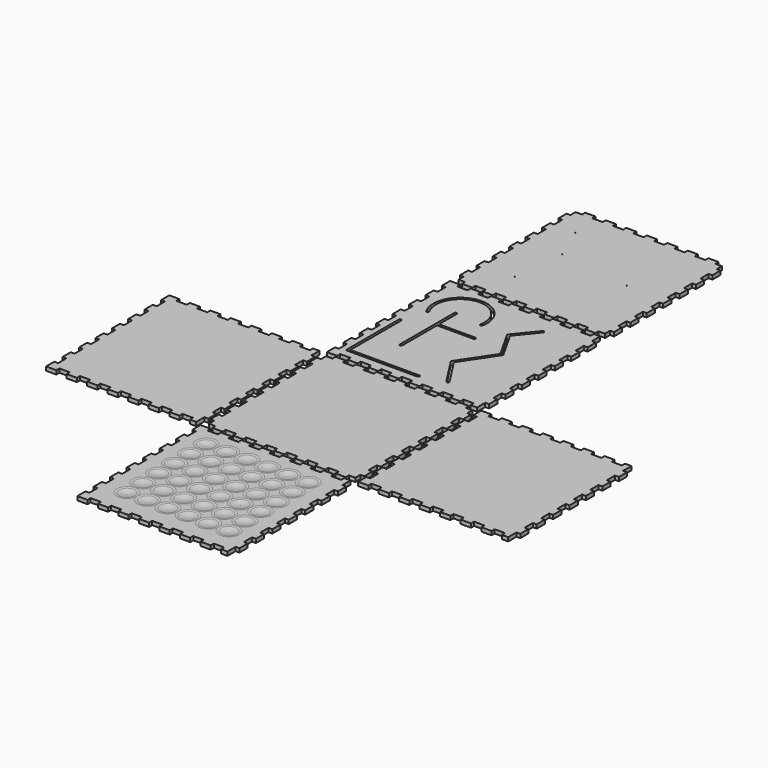
from build123d import *

# Parameters (mm, degrees)
F1_DEPTH = 19.05
F3_DEPTH = 19.051
F4_R     = 44.1721582368
F5_DEPTH = 6.35
F7_R     = 45.72
F8_R     = 1.27
F9_DEPTH = 19.051


# Not quite as in the source:
# - a fillet or chamfer that OpenCascade refuses, or shapes differently, is made with other operations: its cross-section is extruded or revolved along the edge and cut away or added
# - a feature names something its author has since deleted; it is built from what else it names


with BuildPart() as f1:
    # F0 (on Top) → F1 (new body)
    with BuildSketch(Plane.XY):
        Polygon((-361.9498222, 827.8001224), (-361.9498222, 796.0501224), (-330.1998222, 796.0501224), (-330.1998222, 777.0001224), (-279.3998222, 777.0001224), (-279.3998222, 796.0501224), (-228.5998222, 796.0501224), (-228.5998222, 777.0001224), (-177.7998222, 777.0001224), (-177.7998222, 796.0501224), (-126.9998222, 796.0501224), (-126.9998222, 777.0001224), (-76.1998222, 777.0001224), (-76.1998222, 796.0501224), (-25.3998222, 796.0501224), (-25.3998222, 777.0001224), (25.4001778, 777.0001224), (25.4001778, 796.0501224), (76.2001778, 796.0501224), (76.2001778, 777.0001224), (127.0001778, 777.0001224), (127.0001778, 796.0501224), (177.8001778, 796.0501224), (177.8001778, 777.0001224), (228.6001778, 777.0001224), (228.6001778, 796.0501224), (279.4001778, 796.0501224), (279.4001778, 777.0001224), (330.2001778, 777.0001224), (330.2001778, 796.0501224), (361.9501778, 796.0501224), (361.9501778, 827.8001224), (381.0001778, 827.8001224), (381.0001778, 878.6001224), (361.9501778, 878.6001224), (361.9501778, 929.4001224), (381.0001778, 929.4001224), (381.0001778, 980.2001224), (361.9501778, 980.2001224), (361.9501778, 1031.0001224), (381.0001778, 1031.0001224), (381.0001778, 1081.8001224), (361.9501778, 1081.8001224), (361.9501778, 1132.6001224), (381.0001778, 1132.6001224), (381.0001778, 1183.4001224), (361.9501778, 1183.4001224), (361.9501778, 1234.2001224), (381.0001778, 1234.2001224), (381.0001778, 1285.0001224), (361.9501778, 1285.0001224), (361.9501778, 1335.8001224), (381.0001778, 1335.8001224), (381.0001778, 1386.5999446), (361.9501778, 1386.5999446), (361.9501778, 1437.3999446), (381.0001778, 1437.3999446), (381.0001778, 1488.1999446), (361.9501778, 1488.1999446), (361.9501778, 1519.9499446), (330.2001778, 1519.9499446), (330.2001778, 1538.9999446), (279.4001778, 1538.9999446), (279.4001778, 1519.9499446), (228.6001778, 1519.9499446), (228.6001778, 1538.9999446), (177.8001778, 1538.9999446), (177.8001778, 1519.9499446), (127.0001778, 1519.9499446), (127.0001778, 1538.9999446), (76.2001778, 1538.9999446), (76.2001778, 1519.9499446), (25.4001778, 1519.9499446), (25.4001778, 1538.9999446), (-25.3998222, 1538.9999446), (-25.3998222, 1519.9499446), (-76.1998222, 1519.9499446), (-76.1998222, 1538.9999446), (-126.9998222, 1538.9999446), (-126.9998222, 1519.9499446), (-177.7998222, 1519.9499446), (-177.7998222, 1538.9999446), (-228.5998222, 1538.9999446), (-228.5998222, 1519.9499446), (-279.3998222, 1519.9499446), (-279.3998222, 1538.9999446), (-330.1998222, 1538.9999446), (-330.1998222, 1519.9499446), (-361.9498222, 1519.9499446), (-361.9498222, 1488.1999446), (-380.9998222, 1488.1999446), (-380.9998222, 1437.3999446), (-361.9498222, 1437.3999446), (-361.9498222, 1386.5999446), (-380.9998222, 1386.5999446), (-380.9998222, 1335.8001224), (-361.9498222, 1335.8001224), (-361.9498222, 1285.0001224), (-380.9998222, 1285.0001224), (-380.9998222, 1234.2001224), (-361.9498222, 1234.2001224), (-361.9498222, 1183.4001224), (-380.9998222, 1183.4001224), (-380.9998222, 1132.6001224), (-361.9498222, 1132.6001224), (-361.9498222, 1081.8001224), (-380.9998222, 1081.8001224), (-380.9998222, 1031.0001224), (-361.9498222, 1031.0001224), (-361.9498222, 980.2001224), (-380.9998222, 980.2001224), (-380.9998222, 929.4001224), (-361.9498222, 929.4001224), (-361.9498222, 878.6001224), (-380.9998222, 878.6001224), (-380.9998222, 827.8001224), align=None)
    extrude(amount=F1_DEPTH)

    # F8 (on face) → F9 (cut, through all)
    with BuildSketch(Plane.XY.offset(19.05)):
        with Locations((134.9240541458, 1376.1035203934)):
            Circle(F8_R)
        with Locations((0, 1345.3280925751)):
            Circle(F8_R)
        with Locations((178.3542633057, 1161.1238718033)):
            Circle(F8_R)
        with Locations((0, 1011.2895965576)):
            Circle(F8_R)
        with Locations((147.9531228542, 922.2576618195)):
            Circle(F8_R)
        with Locations((-208.1746906042, 950.4873156548)):
            Circle(F8_R)
        with Locations((-182.1165829897, 1211.0686302185)):
            Circle(F8_R)
        with Locations((-255.9479475021, 1384.7895860672)):
            Circle(F8_R)
    extrude(amount=-F9_DEPTH, mode=Mode.SUBTRACT)


with BuildPart() as f1b:
    # F0 (on Top) → F1, piece 2 (new body)
    with BuildSketch(Plane.XY):
        Polygon((-380.9998222, 55.799863), (-380.9998222, 4.999863), (-330.1998222, 4.999863), (-330.1998222, 24.049863), (-279.3998222, 24.049863), (-279.3998222, 4.999863), (-228.5998222, 4.999863), (-228.5998222, 24.049863), (-177.7998222, 24.049863), (-177.7998222, 4.999863), (-126.9998222, 4.999863), (-126.9998222, 24.049863), (-76.1998222, 24.049863), (-76.1998222, 4.999863), (-25.3998222, 4.999863), (-25.3998222, 24.049863), (25.4001778, 24.049863), (25.4001778, 4.999863), (76.2001778, 4.999863), (76.2001778, 24.049863), (127.0001778, 24.049863), (127.0001778, 4.999863), (177.8001778, 4.999863), (177.8001778, 24.049863), (228.6001778, 24.049863), (228.6001778, 4.999863), (279.4001778, 4.999863), (279.4001778, 24.049863), (330.2001778, 24.049863), (330.2001778, 4.999863), (361.9501778, 4.999863), (361.9501778, 55.799863), (381.0001778, 55.799863), (381.0001778, 106.599863), (361.9501778, 106.599863), (361.9501778, 157.399863), (381.0001778, 157.399863), (381.0001778, 208.199863), (361.9501778, 208.199863), (361.9501778, 258.999863), (381.0001778, 258.999863), (381.0001778, 309.799863), (361.9501778, 309.799863), (361.9501778, 360.599863), (381.0001778, 360.599863), (381.0001778, 411.399863), (361.9501778, 411.399863), (361.9501778, 462.199863), (381.0001778, 462.199863), (381.0001778, 512.999863), (361.9501778, 512.999863), (361.9501778, 563.799863), (381.0001778, 563.799863), (381.0001778, 614.599863), (361.9501778, 614.599863), (361.9501778, 665.399863), (381.0001778, 665.399863), (381.0001778, 716.199863), (361.9501778, 716.199863), (361.9501778, 766.999863), (330.2001778, 766.999863), (330.2001778, 747.949863), (279.4001778, 747.949863), (279.4001778, 766.999863), (228.6001778, 766.999863), (228.6001778, 747.949863), (177.8001778, 747.949863), (177.8001778, 766.999863), (127.0001778, 766.999863), (127.0001778, 747.949863), (76.2001778, 747.949863), (76.2001778, 766.999863), (25.4001778, 766.999863), (25.4001778, 747.949863), (-25.3998222, 747.949863), (-25.3998222, 766.999863), (-76.1998222, 766.999863), (-76.1998222, 747.949863), (-126.9998222, 747.949863), (-126.9998222, 766.999863), (-177.7998222, 766.999863), (-177.7998222, 747.949863), (-228.5998222, 747.949863), (-228.5998222, 766.999863), (-279.3998222, 766.999863), (-279.3998222, 747.949863), (-330.1998222, 747.949863), (-330.1998222, 766.999863), (-380.9998222, 766.999863), (-380.9998222, 716.199863), (-361.9498222, 716.199863), (-361.9498222, 665.399863), (-380.9998222, 665.399863), (-380.9998222, 614.599863), (-361.9498222, 614.599863), (-361.9498222, 563.799863), (-380.9998222, 563.799863), (-380.9998222, 512.999863), (-361.9498222, 512.999863), (-361.9498222, 462.199863), (-380.9998222, 462.199863), (-380.9998222, 411.399863), (-361.9498222, 411.399863), (-361.9498222, 360.599863), (-380.9998222, 360.599863), (-380.9998222, 309.799863), (-361.9498222, 309.799863), (-361.9498222, 258.999863), (-380.9998222, 258.999863), (-380.9998222, 208.199863), (-361.9498222, 208.199863), (-361.9498222, 157.399863), (-380.9998222, 157.399863), (-380.9998222, 106.599863), (-361.9498222, 106.599863), (-361.9498222, 55.799863), align=None)
    extrude(amount=F1_DEPTH)

    # F2 (on face) → F3 (cut, through all)
    with BuildSketch(Plane.XY.offset(19.05)):
        with BuildLine():
            ThreePointArc((-62.1652661042, 556.5676306603), (-57.0850951771, 549.1624390118), (-49.6799035286, 554.2426099389))
            ThreePointArc((-49.6799035286, 554.2426099389), (-202.5908994698, 709.3793812781), (-295.1463453373, 512.1924650246))
            ThreePointArc((-295.1463453373, 512.1924650246), (-286.472473156, 509.8667519336), (-284.1467600649, 518.5406241149))
            ThreePointArc((-284.1467600649, 518.5406241149), (-200.4465361302, 696.8617255124), (-62.1652661042, 556.5676306603))
        make_face()
        with BuildLine():
            ThreePointArc((-188.1111880569, 567.0908093452), (-194.4611880569, 573.4408093452), (-200.8111880569, 567.0908093452))
            Line((-200.8111880569, 567.0908093452), (-200.8111880569, 230.2062213421))
            ThreePointArc((-200.8111880569, 230.2062213421), (-194.4611880569, 223.8562213421), (-188.1111880569, 230.2062213421))
            Line((-188.1111880569, 230.2062213421), (-188.1111880569, 438.3612381458))
            ThreePointArc((-188.1111880569, 438.3612381458), (-186.2513161174, 442.8513662064), (-181.7611880569, 444.7112381458))
            Line((-181.7611880569, 444.7112381458), (-8.0722291023, 444.7112381458))
            ThreePointArc((-8.0722291023, 444.7112381458), (-1.7222291023, 451.0612381458), (-8.0722291023, 457.4112381458))
            Line((-8.0722291023, 457.4112381458), (-181.7611880569, 457.4112381458))
            ThreePointArc((-181.7611880569, 457.4112381458), (-186.2513161174, 459.2711100853), (-188.1111880569, 463.7612381458))
            Line((-188.1111880569, 463.7612381458), (-188.1111880569, 567.0908093452))
        make_face()
        with BuildLine():
            ThreePointArc((74.3827268565, 557.599369663), (72.9860006988, 554.1309041272), (73.7832631078, 550.4777589366))
            Line((73.7832631078, 550.4777589366), (150.3360418995, 414.8064545398))
            ThreePointArc((150.3360418995, 414.8064545398), (151.1510086217, 411.4423647395), (150.080549612, 408.1506496164))
            Line((150.080549612, 408.1506496164), (42.9561615174, 248.3145130608))
            ThreePointArc((42.9561615174, 248.3145130608), (41.8813193365, 244.8399185098), (42.889546248, 241.3454126073))
            Line((42.889546248, 241.3454126073), (133.7060332298, 100.0753492117))
            ThreePointArc((133.7060332298, 100.0753492117), (142.481327422, 98.1676773739), (144.3889992598, 106.9429715661))
            Line((144.3889992598, 106.9429715661), (58.0807610297, 241.2002049335))
            ThreePointArc((58.0807610297, 241.2002049335), (57.0725341182, 244.694710836), (58.1473762991, 248.169305387))
            Line((58.1473762991, 248.169305387), (164.9856205487, 407.5784978311))
            ThreePointArc((164.9856205487, 407.5784978311), (166.0560795584, 410.8702129542), (165.2411128362, 414.2343027546))
            Line((165.2411128362, 414.2343027546), (89.0926311433, 549.1890882265))
            ThreePointArc((89.0926311433, 549.1890882265), (88.2953687343, 552.8422334171), (89.692094892, 556.3106989529))
            Line((89.692094892, 556.3106989529), (169.0112754151, 654.0626005675))
            ThreePointArc((169.0112754151, 654.0626005675), (168.0814742098, 662.994591931), (159.1494828463, 662.0647907257))
            Line((159.1494828463, 662.0647907257), (74.3827268565, 557.599369663))
        make_face()
        with BuildLine():
            ThreePointArc((-321.2252173901, 391.1857306957), (-327.5752173901, 397.5357306957), (-333.9252173901, 391.1857306957))
            Line((-333.9252173901, 391.1857306957), (-333.9252173901, 69.2238254309))
            ThreePointArc((-333.9252173901, 69.2238254309), (-332.0653454506, 64.7336973703), (-327.5752173901, 62.8738254309))
            Line((-327.5752173901, 62.8738254309), (20.3780308366, 62.8738254309))
            ThreePointArc((20.3780308366, 62.8738254309), (26.7280308366, 69.2238254309), (20.3780308366, 75.5738254309))
            Line((20.3780308366, 75.5738254309), (-321.2252173901, 75.5738254309))
            Line((-321.2252173901, 75.5738254309), (-321.2252173901, 391.1857306957))
        make_face()
    extrude(amount=-F3_DEPTH, mode=Mode.SUBTRACT)


with BuildPart() as f1c:
    # F0 (on Top) → F1, piece 3 (new body)
    with BuildSketch(Plane.XY):
        Polygon((-361.9498222, -716.199863), (-361.9498222, -747.949863), (-330.1998222, -747.949863), (-330.1998222, -766.999863), (-279.3998222, -766.999863), (-279.3998222, -747.949863), (-228.5998222, -747.949863), (-228.5998222, -766.999863), (-177.7998222, -766.999863), (-177.7998222, -747.949863), (-126.9998222, -747.949863), (-126.9998222, -766.999863), (-76.1998222, -766.999863), (-76.1998222, -747.949863), (-25.3998222, -747.949863), (-25.3998222, -766.999863), (25.4001778, -766.999863), (25.4001778, -747.949863), (76.2001778, -747.949863), (76.2001778, -766.999863), (127.0001778, -766.999863), (127.0001778, -747.949863), (177.8001778, -747.949863), (177.8001778, -766.999863), (228.6001778, -766.999863), (228.6001778, -747.949863), (279.4001778, -747.949863), (279.4001778, -766.999863), (330.2001778, -766.999863), (330.2001778, -747.949863), (361.9501778, -747.949863), (361.9501778, -716.199863), (381.0001778, -716.199863), (381.0001778, -665.399863), (361.9501778, -665.399863), (361.9501778, -614.599863), (381.0001778, -614.599863), (381.0001778, -563.799863), (361.9501778, -563.799863), (361.9501778, -512.999863), (381.0001778, -512.999863), (381.0001778, -462.199863), (361.9501778, -462.199863), (361.9501778, -411.399863), (381.0001778, -411.399863), (381.0001778, -360.599863), (361.9501778, -360.599863), (361.9501778, -309.799863), (381.0001778, -309.799863), (381.0001778, -258.999863), (361.9501778, -258.999863), (361.9501778, -208.199863), (381.0001778, -208.199863), (381.0001778, -157.399863), (361.9501778, -157.399863), (361.9501778, -106.599863), (381.0001778, -106.599863), (381.0001778, -55.799863), (361.9501778, -55.799863), (361.9501778, -24.049863), (330.2001778, -24.049863), (330.2001778, -4.999863), (279.4001778, -4.999863), (279.4001778, -24.049863), (228.6001778, -24.049863), (228.6001778, -4.999863), (177.8001778, -4.999863), (177.8001778, -24.049863), (127.0001778, -24.049863), (127.0001778, -4.999863), (76.2001778, -4.999863), (76.2001778, -24.049863), (25.4001778, -24.049863), (25.4001778, -4.999863), (-25.3998222, -4.999863), (-25.3998222, -24.049863), (-76.1998222, -24.049863), (-76.1998222, -4.999863), (-126.9998222, -4.999863), (-126.9998222, -24.049863), (-177.7998222, -24.049863), (-177.7998222, -4.999863), (-228.5998222, -4.999863), (-228.5998222, -24.049863), (-279.3998222, -24.049863), (-279.3998222, -4.999863), (-330.1998222, -4.999863), (-330.1998222, -24.049863), (-361.9498222, -24.049863), (-361.9498222, -55.799863), (-380.9998222, -55.799863), (-380.9998222, -106.599863), (-361.9498222, -106.599863), (-361.9498222, -157.399863), (-380.9998222, -157.399863), (-380.9998222, -208.199863), (-361.9498222, -208.199863), (-361.9498222, -258.999863), (-380.9998222, -258.999863), (-380.9998222, -309.799863), (-361.9498222, -309.799863), (-361.9498222, -360.599863), (-380.9998222, -360.599863), (-380.9998222, -411.399863), (-361.9498222, -411.399863), (-361.9498222, -462.199863), (-380.9998222, -462.199863), (-380.9998222, -512.999863), (-361.9498222, -512.999863), (-361.9498222, -563.799863), (-380.9998222, -563.799863), (-380.9998222, -614.599863), (-361.9498222, -614.599863), (-361.9498222, -665.399863), (-380.9998222, -665.399863), (-380.9998222, -716.199863), align=None)
    extrude(amount=F1_DEPTH)


with BuildPart() as f1d:
    # F0 (on Top) → F1, piece 4 (new body)
    with BuildSketch(Plane.XY):
        Polygon((390.9999038, -716.199863), (390.9999038, -766.999863), (441.7999038, -766.999863), (441.7999038, -747.949863), (492.5999038, -747.949863), (492.5999038, -766.999863), (543.3999038, -766.999863), (543.3999038, -747.949863), (594.1999038, -747.949863), (594.1999038, -766.999863), (644.9999038, -766.999863), (644.9999038, -747.949863), (695.7999038, -747.949863), (695.7999038, -766.999863), (746.5999038, -766.999863), (746.5999038, -747.949863), (797.3999038, -747.949863), (797.3999038, -766.999863), (848.1999038, -766.999863), (848.1999038, -747.949863), (898.9999038, -747.949863), (898.9999038, -766.999863), (949.7999038, -766.999863), (949.7999038, -747.949863), (1000.5999038, -747.949863), (1000.5999038, -766.999863), (1051.3999038, -766.999863), (1051.3999038, -747.949863), (1102.1999038, -747.949863), (1102.1999038, -766.999863), (1133.9499038, -766.999863), (1133.9499038, -716.199863), (1152.9999038, -716.199863), (1152.9999038, -665.399863), (1133.9499038, -665.399863), (1133.9499038, -614.599863), (1152.9999038, -614.599863), (1152.9999038, -563.799863), (1133.9499038, -563.799863), (1133.9499038, -512.999863), (1152.9999038, -512.999863), (1152.9999038, -462.199863), (1133.9499038, -462.199863), (1133.9499038, -411.399863), (1152.9999038, -411.399863), (1152.9999038, -360.599863), (1133.9499038, -360.599863), (1133.9499038, -309.799863), (1152.9999038, -309.799863), (1152.9999038, -258.999863), (1133.9499038, -258.999863), (1133.9499038, -208.199863), (1152.9999038, -208.199863), (1152.9999038, -157.399863), (1133.9499038, -157.399863), (1133.9499038, -106.599863), (1152.9999038, -106.599863), (1152.9999038, -55.799863), (1133.9499038, -55.799863), (1133.9499038, -4.999863), (1102.1999038, -4.999863), (1102.1999038, -24.049863), (1051.3999038, -24.049863), (1051.3999038, -4.999863), (1000.5999038, -4.999863), (1000.5999038, -24.049863), (949.7999038, -24.049863), (949.7999038, -4.999863), (898.9999038, -4.999863), (898.9999038, -24.049863), (848.1999038, -24.049863), (848.1999038, -4.999863), (797.3999038, -4.999863), (797.3999038, -24.049863), (746.5999038, -24.049863), (746.5999038, -4.999863), (695.7999038, -4.999863), (695.7999038, -24.049863), (644.9999038, -24.049863), (644.9999038, -4.999863), (594.1999038, -4.999863), (594.1999038, -24.049863), (543.3999038, -24.049863), (543.3999038, -4.999863), (492.5999038, -4.999863), (492.5999038, -24.049863), (441.7999038, -24.049863), (441.7999038, -4.999863), (390.9999038, -4.999863), (390.9999038, -55.799863), (410.0499038, -55.799863), (410.0499038, -106.599863), (390.9999038, -106.599863), (390.9999038, -157.399863), (410.0499038, -157.399863), (410.0499038, -208.199863), (390.9999038, -208.199863), (390.9999038, -258.999863), (410.0499038, -258.999863), (410.0499038, -309.799863), (390.9999038, -309.799863), (390.9999038, -360.599863), (410.0499038, -360.599863), (410.0499038, -411.399863), (390.9999038, -411.399863), (390.9999038, -462.199863), (410.0499038, -462.199863), (410.0499038, -512.999863), (390.9999038, -512.999863), (390.9999038, -563.799863), (410.0499038, -563.799863), (410.0499038, -614.599863), (390.9999038, -614.599863), (390.9999038, -665.399863), (410.0499038, -665.399863), (410.0499038, -716.199863), align=None)
    extrude(amount=F1_DEPTH)


with BuildPart() as f1e:
    # F0 (on Top) → F1, piece 5 (new body)
    with BuildSketch(Plane.XY):
        Polygon((-1152.9999038, -716.199863), (-1152.9999038, -766.999863), (-1102.1999038, -766.999863), (-1102.1999038, -747.949863), (-1051.3999038, -747.949863), (-1051.3999038, -766.999863), (-1000.5999038, -766.999863), (-1000.5999038, -747.949863), (-949.7999038, -747.949863), (-949.7999038, -766.999863), (-898.9999038, -766.999863), (-898.9999038, -747.949863), (-848.1999038, -747.949863), (-848.1999038, -766.999863), (-797.4002594, -766.999863), (-797.4002594, -747.949863), (-746.6002594, -747.949863), (-746.6002594, -766.999863), (-695.8002594, -766.999863), (-695.8002594, -747.949863), (-645.0002594, -747.949863), (-645.0002594, -766.999863), (-594.2002594, -766.999863), (-594.2002594, -747.949863), (-543.4002594, -747.949863), (-543.4002594, -766.999863), (-492.6002594, -766.999863), (-492.6002594, -747.949863), (-441.8002594, -747.949863), (-441.8002594, -766.999863), (-410.0502594, -766.999863), (-410.0502594, -716.199863), (-391.0002594, -716.199863), (-391.0002594, -665.399863), (-410.0502594, -665.399863), (-410.0502594, -614.599863), (-391.0002594, -614.599863), (-391.0002594, -563.799863), (-410.0502594, -563.799863), (-410.0502594, -512.999863), (-391.0002594, -512.999863), (-391.0002594, -462.199863), (-410.0502594, -462.199863), (-410.0502594, -411.399863), (-391.0002594, -411.399863), (-391.0002594, -360.599863), (-410.0502594, -360.599863), (-410.0502594, -309.799863), (-391.0002594, -309.799863), (-391.0002594, -258.999863), (-410.0502594, -258.999863), (-410.0502594, -208.199863), (-391.0002594, -208.199863), (-391.0002594, -157.399863), (-410.0502594, -157.399863), (-410.0502594, -106.599863), (-391.0002594, -106.599863), (-391.0002594, -55.799863), (-410.0502594, -55.799863), (-410.0502594, -4.999863), (-441.8002594, -4.999863), (-441.8002594, -24.049863), (-492.6002594, -24.049863), (-492.6002594, -4.999863), (-543.4002594, -4.999863), (-543.4002594, -24.049863), (-594.2002594, -24.049863), (-594.2002594, -4.999863), (-645.0002594, -4.999863), (-645.0002594, -24.049863), (-695.8002594, -24.049863), (-695.8002594, -4.999863), (-746.6002594, -4.999863), (-746.6002594, -24.049863), (-797.4002594, -24.049863), (-797.4002594, -4.999863), (-848.1999038, -4.999863), (-848.1999038, -24.049863), (-898.9999038, -24.049863), (-898.9999038, -4.999863), (-949.7999038, -4.999863), (-949.7999038, -24.049863), (-1000.5999038, -24.049863), (-1000.5999038, -4.999863), (-1051.3999038, -4.999863), (-1051.3999038, -24.049863), (-1102.1999038, -24.049863), (-1102.1999038, -4.999863), (-1152.9999038, -4.999863), (-1152.9999038, -55.799863), (-1133.9499038, -55.799863), (-1133.9499038, -106.599863), (-1152.9999038, -106.599863), (-1152.9999038, -157.399863), (-1133.9499038, -157.399863), (-1133.9499038, -208.199863), (-1152.9999038, -208.199863), (-1152.9999038, -258.999863), (-1133.9499038, -258.999863), (-1133.9499038, -309.799863), (-1152.9999038, -309.799863), (-1152.9999038, -360.599863), (-1133.9499038, -360.599863), (-1133.9499038, -411.399863), (-1152.9999038, -411.399863), (-1152.9999038, -462.199863), (-1133.9499038, -462.199863), (-1133.9499038, -512.999863), (-1152.9999038, -512.999863), (-1152.9999038, -563.799863), (-1133.9499038, -563.799863), (-1133.9499038, -614.599863), (-1152.9999038, -614.599863), (-1152.9999038, -665.399863), (-1133.9499038, -665.399863), (-1133.9499038, -716.199863), align=None)
    extrude(amount=F1_DEPTH)


with BuildPart() as f1f:
    # F0 (on Top) → F1, piece 6 (new body)
    with BuildSketch(Plane.XY):
        Polygon((-380.9998222, -1488.1999446), (-380.9998222, -1538.9999446), (-330.1998222, -1538.9999446), (-330.1998222, -1519.9499446), (-279.3998222, -1519.9499446), (-279.3998222, -1538.9999446), (-228.5998222, -1538.9999446), (-228.5998222, -1519.9499446), (-177.7998222, -1519.9499446), (-177.7998222, -1538.9999446), (-126.9998222, -1538.9999446), (-126.9998222, -1519.9499446), (-76.1998222, -1519.9499446), (-76.1998222, -1538.9999446), (-25.3998222, -1538.9999446), (-25.3998222, -1519.9499446), (25.4001778, -1519.9499446), (25.4001778, -1538.9999446), (76.2001778, -1538.9999446), (76.2001778, -1519.9499446), (127.0001778, -1519.9499446), (127.0001778, -1538.9999446), (177.8001778, -1538.9999446), (177.8001778, -1519.9499446), (228.6001778, -1519.9499446), (228.6001778, -1538.9999446), (279.4001778, -1538.9999446), (279.4001778, -1519.9499446), (330.2001778, -1519.9499446), (330.2001778, -1538.9999446), (361.9501778, -1538.9999446), (361.9501778, -1488.1999446), (381.0001778, -1488.1999446), (381.0001778, -1437.3999446), (361.9501778, -1437.3999446), (361.9501778, -1386.5999446), (381.0001778, -1386.5999446), (381.0001778, -1335.7999446), (361.9501778, -1335.7999446), (361.9501778, -1284.9999446), (381.0001778, -1284.9999446), (381.0001778, -1234.1999446), (361.9501778, -1234.1999446), (361.9501778, -1183.4003002), (381.0001778, -1183.4003002), (381.0001778, -1132.6003002), (361.9501778, -1132.6003002), (361.9501778, -1081.8003002), (381.0001778, -1081.8003002), (381.0001778, -1031.0003002), (361.9501778, -1031.0003002), (361.9501778, -980.2003002), (381.0001778, -980.2003002), (381.0001778, -929.4003002), (361.9501778, -929.4003002), (361.9501778, -878.6003002), (381.0001778, -878.6003002), (381.0001778, -827.8003002), (361.9501778, -827.8003002), (361.9501778, -777.0003002), (330.2001778, -777.0003002), (330.2001778, -796.0503002), (279.4001778, -796.0503002), (279.4001778, -777.0003002), (228.6001778, -777.0003002), (228.6001778, -796.0503002), (177.8001778, -796.0503002), (177.8001778, -777.0003002), (127.0001778, -777.0003002), (127.0001778, -796.0503002), (76.2001778, -796.0503002), (76.2001778, -777.0003002), (25.4001778, -777.0003002), (25.4001778, -796.0503002), (-25.3998222, -796.0503002), (-25.3998222, -777.0003002), (-76.1998222, -777.0003002), (-76.1998222, -796.0503002), (-126.9998222, -796.0503002), (-126.9998222, -777.0003002), (-177.7998222, -777.0003002), (-177.7998222, -796.0503002), (-228.5998222, -796.0503002), (-228.5998222, -777.0003002), (-279.3998222, -777.0003002), (-279.3998222, -796.0503002), (-330.1998222, -796.0503002), (-330.1998222, -777.0003002), (-380.9998222, -777.0003002), (-380.9998222, -827.8003002), (-361.9498222, -827.8003002), (-361.9498222, -878.6003002), (-380.9998222, -878.6003002), (-380.9998222, -929.4003002), (-361.9498222, -929.4003002), (-361.9498222, -980.2003002), (-380.9998222, -980.2003002), (-380.9998222, -1031.0003002), (-361.9498222, -1031.0003002), (-361.9498222, -1081.8003002), (-380.9998222, -1081.8003002), (-380.9998222, -1132.6003002), (-361.9498222, -1132.6003002), (-361.9498222, -1183.4003002), (-380.9998222, -1183.4003002), (-380.9998222, -1234.1999446), (-361.9498222, -1234.1999446), (-361.9498222, -1284.9999446), (-380.9998222, -1284.9999446), (-380.9998222, -1335.7999446), (-361.9498222, -1335.7999446), (-361.9498222, -1386.5999446), (-380.9998222, -1386.5999446), (-380.9998222, -1437.3999446), (-361.9498222, -1437.3999446), (-361.9498222, -1488.1999446), align=None)
    extrude(amount=F1_DEPTH)

    # F4 (on face) → F5 (cut)
    with BuildSketch(Plane.XY.offset(19.05)):
        with Locations((-54.9763494369, -1092.6421843415)):
            Circle(F4_R)
        with Locations((-156.5725402639, -1091.7624062665)):
            Circle(F4_R)
        with Locations((-258.1687310908, -1090.8826281916)):
            Circle(F4_R)
        with Locations((-261.0486020433, -989.3234516328)):
            Circle(F4_R)
        with Locations((-159.4524112164, -990.2032297077)):
            Circle(F4_R)
        with Locations((-57.8562203894, -991.0830077827)):
            Circle(F4_R)
        with Locations((-263.9284729958, -887.764275074)):
            Circle(F4_R)
        with Locations((-162.3322821688, -888.644053149)):
            Circle(F4_R)
        with Locations((-60.7360913419, -889.5238312239)):
            Circle(F4_R)
        with Locations((40.860099485, -890.4036092989)):
            Circle(F4_R)
        with Locations((43.7399704375, -991.9627858576)):
            Circle(F4_R)
        with Locations((46.61984139, -1093.5219624164)):
            Circle(F4_R)
        with Locations((148.2160322169, -1094.4017404914)):
            Circle(F4_R)
        with Locations((145.3361612644, -992.8425639326)):
            Circle(F4_R)
        with Locations((142.4562903119, -891.2833873738)):
            Circle(F4_R)
        with Locations((244.0524811388, -892.1631654488)):
            Circle(F4_R)
        with Locations((246.9323520913, -993.7223420075)):
            Circle(F4_R)
        with Locations((249.8122230438, -1095.2815185663)):
            Circle(F4_R)
        with Locations((-52.0964784845, -1194.2013609002)):
            Circle(F4_R)
        with Locations((-153.6926693114, -1193.3215828253)):
            Circle(F4_R)
        with Locations((-255.2888601383, -1192.4418047503)):
            Circle(F4_R)
        with Locations((-252.4089891858, -1294.0009813091)):
            Circle(F4_R)
        with Locations((-150.8127983589, -1294.8807593841)):
            Circle(F4_R)
        with Locations((-49.216607532, -1295.760537459)):
            Circle(F4_R)
        with Locations((49.4997123425, -1195.0811389752)):
            Circle(F4_R)
        with Locations((151.0959031694, -1195.9609170501)):
            Circle(F4_R)
        with Locations((252.6920939963, -1196.8406951251)):
            Circle(F4_R)
        with Locations((255.5719649488, -1298.3998716839)):
            Circle(F4_R)
        with Locations((153.9757741219, -1297.5200936089)):
            Circle(F4_R)
        with Locations((52.379583295, -1296.640315534)):
            Circle(F4_R)
        with Locations((55.2594542474, -1398.1994920927)):
            Circle(F4_R)
        with Locations((156.8556450744, -1399.0792701677)):
            Circle(F4_R)
        with Locations((258.4518359013, -1399.9590482426)):
            Circle(F4_R)
        with Locations((-46.3367365795, -1397.3197140178)):
            Circle(F4_R)
        with Locations((-147.9329274064, -1396.4399359428)):
            Circle(F4_R)
        with Locations((-249.5291182333, -1395.5601578679)):
            Circle(F4_R)
    extrude(amount=-F5_DEPTH, mode=Mode.SUBTRACT)

    # F6: fillet of radius 154.94 on 36 edges, made by hand

    # F6_s1 → F6_t2 (revolve)
    with BuildSketch(Plane.XZ.offset(887.764275074)):
        with BuildLine():
            ThreePointArc((-219.7563147589, 19.05), (-241.4790587636, 14.2957170939), (-263.6586552432, 12.7))
            Line((-263.6586552432, 12.7), (-219.7563147589, 12.7))
            Line((-219.7563147589, 12.7), (-219.7563147589, 19.05))
        make_face()
    revolve(axis=Axis((-263.9284729958, -887.764275074, 12.7), (0, 0, 1)))

    # F6_s3 → F6_t4 (revolve)
    with BuildSketch(Plane.XZ.offset(989.3234516328)):
        with BuildLine():
            ThreePointArc((-216.8764438064, 19.05), (-238.5991878111, 14.2957170939), (-260.7787842907, 12.7))
            Line((-260.7787842907, 12.7), (-216.8764438064, 12.7))
            Line((-216.8764438064, 12.7), (-216.8764438064, 19.05))
        make_face()
    revolve(axis=Axis((-261.0486020433, -989.3234516328, 12.7), (0, 0, 1)))

    # F6_s5 → F6_t6 (revolve)
    with BuildSketch(Plane.XZ.offset(888.644053149)):
        with BuildLine():
            ThreePointArc((-118.160123932, 19.05), (-139.8828679367, 14.2957170939), (-162.0624644163, 12.7))
            Line((-162.0624644163, 12.7), (-118.160123932, 12.7))
            Line((-118.160123932, 12.7), (-118.160123932, 19.05))
        make_face()
    revolve(axis=Axis((-162.3322821688, -888.644053149, 12.7), (0, 0, 1)))

    # F6_s7 → F6_t8 (revolve)
    with BuildSketch(Plane.XZ.offset(990.2032297077)):
        with BuildLine():
            ThreePointArc((-115.2802529795, 19.05), (-137.0029969842, 14.2957170939), (-159.1825934638, 12.7))
            Line((-159.1825934638, 12.7), (-115.2802529795, 12.7))
            Line((-115.2802529795, 12.7), (-115.2802529795, 19.05))
        make_face()
    revolve(axis=Axis((-159.4524112164, -990.2032297077, 12.7), (0, 0, 1)))

    # F6_s9 → F6_t10 (revolve)
    with BuildSketch(Plane.XZ.offset(991.0830077827)):
        with BuildLine():
            ThreePointArc((-13.6840621526, 19.05), (-35.4068061573, 14.2957170939), (-57.5864026369, 12.7))
            Line((-57.5864026369, 12.7), (-13.6840621526, 12.7))
            Line((-13.6840621526, 12.7), (-13.6840621526, 19.05))
        make_face()
    revolve(axis=Axis((-57.8562203894, -991.0830077827, 12.7), (0, 0, 1)))

    # F6_s11 → F6_t12 (revolve)
    with BuildSketch(Plane.XZ.offset(889.5238312239)):
        with BuildLine():
            ThreePointArc((-16.5639331051, 19.05), (-38.2866771097, 14.2957170939), (-60.4662735894, 12.7))
            Line((-60.4662735894, 12.7), (-16.5639331051, 12.7))
            Line((-16.5639331051, 12.7), (-16.5639331051, 19.05))
        make_face()
    revolve(axis=Axis((-60.7360913419, -889.5238312239, 12.7), (0, 0, 1)))

    # F6_s13 → F6_t14 (revolve)
    with BuildSketch(Plane.XZ.offset(890.4036092989)):
        with BuildLine():
            ThreePointArc((85.0322577218, 19.05), (63.3095137172, 14.2957170939), (41.1299172375, 12.7))
            Line((41.1299172375, 12.7), (85.0322577218, 12.7))
            Line((85.0322577218, 12.7), (85.0322577218, 19.05))
        make_face()
    revolve(axis=Axis((40.860099485, -890.4036092989, 12.7), (0, 0, 1)))

    # F6_s15 → F6_t16 (revolve)
    with BuildSketch(Plane.XZ.offset(991.9627858576)):
        with BuildLine():
            ThreePointArc((87.9121286743, 19.05), (66.1893846697, 14.2957170939), (44.00978819, 12.7))
            Line((44.00978819, 12.7), (87.9121286743, 12.7))
            Line((87.9121286743, 12.7), (87.9121286743, 19.05))
        make_face()
    revolve(axis=Axis((43.7399704375, -991.9627858576, 12.7), (0, 0, 1)))

    # F6_s17 → F6_t18 (revolve)
    with BuildSketch(Plane.XZ.offset(891.2833873738)):
        with BuildLine():
            ThreePointArc((186.6284485487, 19.05), (164.9057045441, 14.2957170939), (142.7261080644, 12.7))
            Line((142.7261080644, 12.7), (186.6284485487, 12.7))
            Line((186.6284485487, 12.7), (186.6284485487, 19.05))
        make_face()
    revolve(axis=Axis((142.4562903119, -891.2833873738, 12.7), (0, 0, 1)))

    # F6_s19 → F6_t20 (revolve)
    with BuildSketch(Plane.XZ.offset(992.8425639326)):
        with BuildLine():
            ThreePointArc((189.5083195012, 19.05), (167.7855754966, 14.2957170939), (145.6059790169, 12.7))
            Line((145.6059790169, 12.7), (189.5083195012, 12.7))
            Line((189.5083195012, 12.7), (189.5083195012, 19.05))
        make_face()
    revolve(axis=Axis((145.3361612644, -992.8425639326, 12.7), (0, 0, 1)))

    # F6_s21 → F6_t22 (revolve)
    with BuildSketch(Plane.XZ.offset(1094.4017404914)):
        with BuildLine():
            ThreePointArc((192.3881904537, 19.05), (170.6654464491, 14.2957170939), (148.4858499694, 12.7))
            Line((148.4858499694, 12.7), (192.3881904537, 12.7))
            Line((192.3881904537, 12.7), (192.3881904537, 19.05))
        make_face()
    revolve(axis=Axis((148.2160322169, -1094.4017404914, 12.7), (0, 0, 1)))

    # F6_s23 → F6_t24 (revolve)
    with BuildSketch(Plane.XZ.offset(1093.5219624164)):
        with BuildLine():
            ThreePointArc((90.7919996268, 19.05), (69.0692556221, 14.2957170939), (46.8896591425, 12.7))
            Line((46.8896591425, 12.7), (90.7919996268, 12.7))
            Line((90.7919996268, 12.7), (90.7919996268, 19.05))
        make_face()
    revolve(axis=Axis((46.61984139, -1093.5219624164, 12.7), (0, 0, 1)))

    # F6_s25 → F6_t26 (revolve)
    with BuildSketch(Plane.XZ.offset(1092.6421843415)):
        with BuildLine():
            ThreePointArc((-10.8041912001, 19.05), (-32.5269352048, 14.2957170939), (-54.7065316844, 12.7))
            Line((-54.7065316844, 12.7), (-10.8041912001, 12.7))
            Line((-10.8041912001, 12.7), (-10.8041912001, 19.05))
        make_face()
    revolve(axis=Axis((-54.9763494369, -1092.6421843415, 12.7), (0, 0, 1)))

    # F6_s27 → F6_t28 (revolve)
    with BuildSketch(Plane.XZ.offset(1091.7624062665)):
        with BuildLine():
            ThreePointArc((-112.400382027, 19.05), (-134.1231260317, 14.2957170939), (-156.3027225113, 12.7))
            Line((-156.3027225113, 12.7), (-112.400382027, 12.7))
            Line((-112.400382027, 12.7), (-112.400382027, 19.05))
        make_face()
    revolve(axis=Axis((-156.5725402639, -1091.7624062665, 12.7), (0, 0, 1)))

    # F6_s29 → F6_t30 (revolve)
    with BuildSketch(Plane.XZ.offset(1090.8826281916)):
        with BuildLine():
            ThreePointArc((-213.9965728539, 19.05), (-235.7193168586, 14.2957170939), (-257.8989133382, 12.7))
            Line((-257.8989133382, 12.7), (-213.9965728539, 12.7))
            Line((-213.9965728539, 12.7), (-213.9965728539, 19.05))
        make_face()
    revolve(axis=Axis((-258.1687310908, -1090.8826281916, 12.7), (0, 0, 1)))

    # F6_s31 → F6_t32 (revolve)
    with BuildSketch(Plane.XZ.offset(1192.4418047503)):
        with BuildLine():
            ThreePointArc((-211.1167019014, 19.05), (-232.8394459061, 14.2957170939), (-255.0190423857, 12.7))
            Line((-255.0190423857, 12.7), (-211.1167019014, 12.7))
            Line((-211.1167019014, 12.7), (-211.1167019014, 19.05))
        make_face()
    revolve(axis=Axis((-255.2888601383, -1192.4418047503, 12.7), (0, 0, 1)))

    # F6_s33 → F6_t34 (revolve)
    with BuildSketch(Plane.XZ.offset(1193.3215828253)):
        with BuildLine():
            ThreePointArc((-109.5205110745, 19.05), (-131.2432550792, 14.2957170939), (-153.4228515588, 12.7))
            Line((-153.4228515588, 12.7), (-109.5205110745, 12.7))
            Line((-109.5205110745, 12.7), (-109.5205110745, 19.05))
        make_face()
    revolve(axis=Axis((-153.6926693114, -1193.3215828253, 12.7), (0, 0, 1)))

    # F6_s35 → F6_t36 (revolve)
    with BuildSketch(Plane.XZ.offset(1194.2013609002)):
        with BuildLine():
            ThreePointArc((-7.9243202476, 19.05), (-29.6470642523, 14.2957170939), (-51.8266607319, 12.7))
            Line((-51.8266607319, 12.7), (-7.9243202476, 12.7))
            Line((-7.9243202476, 12.7), (-7.9243202476, 19.05))
        make_face()
    revolve(axis=Axis((-52.0964784845, -1194.2013609002, 12.7), (0, 0, 1)))

    # F6_s37 → F6_t38 (revolve)
    with BuildSketch(Plane.XZ.offset(1195.0811389752)):
        with BuildLine():
            ThreePointArc((93.6718705793, 19.05), (71.9491265746, 14.2957170939), (49.769530095, 12.7))
            Line((49.769530095, 12.7), (93.6718705793, 12.7))
            Line((93.6718705793, 12.7), (93.6718705793, 19.05))
        make_face()
    revolve(axis=Axis((49.4997123425, -1195.0811389752, 12.7), (0, 0, 1)))

    # F6_s39 → F6_t40 (revolve)
    with BuildSketch(Plane.XZ.offset(1195.9609170501)):
        with BuildLine():
            ThreePointArc((195.2680614062, 19.05), (173.5453174016, 14.2957170939), (151.3657209219, 12.7))
            Line((151.3657209219, 12.7), (195.2680614062, 12.7))
            Line((195.2680614062, 12.7), (195.2680614062, 19.05))
        make_face()
    revolve(axis=Axis((151.0959031694, -1195.9609170501, 12.7), (0, 0, 1)))

    # F6_s41 → F6_t42 (revolve)
    with BuildSketch(Plane.XZ.offset(1296.640315534)):
        with BuildLine():
            ThreePointArc((96.5517415318, 19.05), (74.8289975271, 14.2957170939), (52.6494010475, 12.7))
            Line((52.6494010475, 12.7), (96.5517415318, 12.7))
            Line((96.5517415318, 12.7), (96.5517415318, 19.05))
        make_face()
    revolve(axis=Axis((52.379583295, -1296.640315534, 12.7), (0, 0, 1)))

    # F6_s43 → F6_t44 (revolve)
    with BuildSketch(Plane.XZ.offset(1295.760537459)):
        with BuildLine():
            ThreePointArc((-5.0444492951, 19.05), (-26.7671932998, 14.2957170939), (-48.9467897794, 12.7))
            Line((-48.9467897794, 12.7), (-5.0444492951, 12.7))
            Line((-5.0444492951, 12.7), (-5.0444492951, 19.05))
        make_face()
    revolve(axis=Axis((-49.216607532, -1295.760537459, 12.7), (0, 0, 1)))

    # F6_s45 → F6_t46 (revolve)
    with BuildSketch(Plane.XZ.offset(1294.8807593841)):
        with BuildLine():
            ThreePointArc((-106.640640122, 19.05), (-128.3633841267, 14.2957170939), (-150.5429806063, 12.7))
            Line((-150.5429806063, 12.7), (-106.640640122, 12.7))
            Line((-106.640640122, 12.7), (-106.640640122, 19.05))
        make_face()
    revolve(axis=Axis((-150.8127983589, -1294.8807593841, 12.7), (0, 0, 1)))

    # F6_s47 → F6_t48 (revolve)
    with BuildSketch(Plane.XZ.offset(1294.0009813091)):
        with BuildLine():
            ThreePointArc((-208.236830949, 19.05), (-229.9595749536, 14.2957170939), (-252.1391714333, 12.7))
            Line((-252.1391714333, 12.7), (-208.236830949, 12.7))
            Line((-208.236830949, 12.7), (-208.236830949, 19.05))
        make_face()
    revolve(axis=Axis((-252.4089891858, -1294.0009813091, 12.7), (0, 0, 1)))

    # F6_s49 → F6_t50 (revolve)
    with BuildSketch(Plane.XZ.offset(1395.5601578679)):
        with BuildLine():
            ThreePointArc((-205.3569599965, 19.05), (-227.0797040011, 14.2957170939), (-249.2593004808, 12.7))
            Line((-249.2593004808, 12.7), (-205.3569599965, 12.7))
            Line((-205.3569599965, 12.7), (-205.3569599965, 19.05))
        make_face()
    revolve(axis=Axis((-249.5291182333, -1395.5601578679, 12.7), (0, 0, 1)))

    # F6_s51 → F6_t52 (revolve)
    with BuildSketch(Plane.XZ.offset(1396.4399359428)):
        with BuildLine():
            ThreePointArc((-103.7607691695, 19.05), (-125.4835131742, 14.2957170939), (-147.6631096539, 12.7))
            Line((-147.6631096539, 12.7), (-103.7607691695, 12.7))
            Line((-103.7607691695, 12.7), (-103.7607691695, 19.05))
        make_face()
    revolve(axis=Axis((-147.9329274064, -1396.4399359428, 12.7), (0, 0, 1)))

    # F6_s53 → F6_t54 (revolve)
    with BuildSketch(Plane.XZ.offset(1397.3197140178)):
        with BuildLine():
            ThreePointArc((-2.1645783426, 19.05), (-23.8873223473, 14.2957170939), (-46.0669188269, 12.7))
            Line((-46.0669188269, 12.7), (-2.1645783426, 12.7))
            Line((-2.1645783426, 12.7), (-2.1645783426, 19.05))
        make_face()
    revolve(axis=Axis((-46.3367365795, -1397.3197140178, 12.7), (0, 0, 1)))

    # F6_s55 → F6_t56 (revolve)
    with BuildSketch(Plane.XZ.offset(1398.1994920927)):
        with BuildLine():
            ThreePointArc((99.4316124843, 19.05), (77.7088684796, 14.2957170939), (55.529272, 12.7))
            Line((55.529272, 12.7), (99.4316124843, 12.7))
            Line((99.4316124843, 12.7), (99.4316124843, 19.05))
        make_face()
    revolve(axis=Axis((55.2594542474, -1398.1994920927, 12.7), (0, 0, 1)))

    # F6_s57 → F6_t58 (revolve)
    with BuildSketch(Plane.XZ.offset(1399.0792701677)):
        with BuildLine():
            ThreePointArc((201.0278033112, 19.05), (179.3050593065, 14.2957170939), (157.1254628269, 12.7))
            Line((157.1254628269, 12.7), (201.0278033112, 12.7))
            Line((201.0278033112, 12.7), (201.0278033112, 19.05))
        make_face()
    revolve(axis=Axis((156.8556450744, -1399.0792701677, 12.7), (0, 0, 1)))

    # F6_s59 → F6_t60 (revolve)
    with BuildSketch(Plane.XZ.offset(1297.5200936089)):
        with BuildLine():
            ThreePointArc((198.1479323587, 19.05), (176.425188354, 14.2957170939), (154.2455918744, 12.7))
            Line((154.2455918744, 12.7), (198.1479323587, 12.7))
            Line((198.1479323587, 12.7), (198.1479323587, 19.05))
        make_face()
    revolve(axis=Axis((153.9757741219, -1297.5200936089, 12.7), (0, 0, 1)))

    # F6_s61 → F6_t62 (revolve)
    with BuildSketch(Plane.XZ.offset(892.1631654488)):
        with BuildLine():
            ThreePointArc((288.2246393757, 19.05), (266.501895371, 14.2957170939), (244.3222988913, 12.7))
            Line((244.3222988913, 12.7), (288.2246393757, 12.7))
            Line((288.2246393757, 12.7), (288.2246393757, 19.05))
        make_face()
    revolve(axis=Axis((244.0524811388, -892.1631654488, 12.7), (0, 0, 1)))

    # F6_s63 → F6_t64 (revolve)
    with BuildSketch(Plane.XZ.offset(993.7223420075)):
        with BuildLine():
            ThreePointArc((291.1045103281, 19.05), (269.3817663235, 14.2957170939), (247.2021698438, 12.7))
            Line((247.2021698438, 12.7), (291.1045103281, 12.7))
            Line((291.1045103281, 12.7), (291.1045103281, 19.05))
        make_face()
    revolve(axis=Axis((246.9323520913, -993.7223420075, 12.7), (0, 0, 1)))

    # F6_s65 → F6_t66 (revolve)
    with BuildSketch(Plane.XZ.offset(1095.2815185663)):
        with BuildLine():
            ThreePointArc((293.9843812806, 19.05), (272.261637276, 14.2957170939), (250.0820407963, 12.7))
            Line((250.0820407963, 12.7), (293.9843812806, 12.7))
            Line((293.9843812806, 12.7), (293.9843812806, 19.05))
        make_face()
    revolve(axis=Axis((249.8122230438, -1095.2815185663, 12.7), (0, 0, 1)))

    # F6_s67 → F6_t68 (revolve)
    with BuildSketch(Plane.XZ.offset(1196.8406951251)):
        with BuildLine():
            ThreePointArc((296.8642522331, 19.05), (275.1415082285, 14.2957170939), (252.9619117488, 12.7))
            Line((252.9619117488, 12.7), (296.8642522331, 12.7))
            Line((296.8642522331, 12.7), (296.8642522331, 19.05))
        make_face()
    revolve(axis=Axis((252.6920939963, -1196.8406951251, 12.7), (0, 0, 1)))

    # F6_s69 → F6_t70 (revolve)
    with BuildSketch(Plane.XZ.offset(1298.3998716839)):
        with BuildLine():
            ThreePointArc((299.7441231856, 19.05), (278.021379181, 14.2957170939), (255.8417827013, 12.7))
            Line((255.8417827013, 12.7), (299.7441231856, 12.7))
            Line((299.7441231856, 12.7), (299.7441231856, 19.05))
        make_face()
    revolve(axis=Axis((255.5719649488, -1298.3998716839, 12.7), (0, 0, 1)))

    # F6_s71 → F6_t72 (revolve)
    with BuildSketch(Plane.XZ.offset(1399.9590482426)):
        with BuildLine():
            ThreePointArc((302.6239941381, 19.05), (280.9012501335, 14.2957170939), (258.7216536538, 12.7))
            Line((258.7216536538, 12.7), (302.6239941381, 12.7))
            Line((302.6239941381, 12.7), (302.6239941381, 19.05))
        make_face()
    revolve(axis=Axis((258.4518359013, -1399.9590482426, 12.7), (0, 0, 1)))

    # F7
    f7_edges = [f1f.edges().sort_by_distance(p)[0] for p in [
        (5.327554, -1195.081139, 19.05),
        (106.923745, -1195.960917, 19.05),
        (170.665446, -1094.40174, 14.295717),
        (147.946214, -1094.40174, 12.7),
        (104.043874, -1094.40174, 19.05),
        (69.069256, -1093.521962, 14.295717),
        (46.350024, -1093.521962, 12.7),
        (2.447683, -1093.521962, 19.05),
        (-99.148508, -1092.642184, 19.05),
        (-134.123126, -1091.762406, 14.295717),
        (-156.842358, -1091.762406, 12.7),
        (-200.744699, -1091.762406, 19.05),
        (-302.340889, -1090.882628, 19.05),
        (-305.22076, -989.323452, 19.05),
        (-308.100631, -887.764275, 19.05),
        (-206.50444, -888.644053, 19.05),
        (-203.624569, -990.20323, 19.05),
        (-104.90825, -889.523831, 19.05),
        (-0.432188, -991.962786, 19.05),
        (-3.312059, -890.403609, 19.05),
        (98.284132, -891.283387, 19.05),
        (-102.028379, -991.083008, 19.05),
        (101.164003, -992.842564, 19.05),
        (205.640065, -1095.281519, 19.05),
        (202.760194, -993.722342, 19.05),
        (199.880323, -892.163165, 19.05),
        (208.519936, -1196.840695, 19.05),
        (211.399807, -1298.399872, 19.05),
        (109.803616, -1297.520094, 19.05),
        (8.207425, -1296.640316, 19.05),
        (-93.388766, -1295.760537, 19.05),
        (-96.268637, -1194.201361, 19.05),
        (-197.864828, -1193.321583, 19.05),
        (-299.461018, -1192.441805, 19.05),
        (-296.581147, -1294.000981, 19.05),
        (-194.984957, -1294.880759, 19.05),
        (-293.701276, -1395.560158, 19.05),
        (-192.105086, -1396.439936, 19.05),
        (-90.508895, -1397.319714, 19.05),
        (11.087296, -1398.199492, 19.05),
        (112.683487, -1399.07927, 19.05),
        (214.279678, -1399.959048, 19.05),
    ]]
    fillet(f7_edges, radius=F7_R)


solid = Compound([f1.part, f1b.part, f1c.part, f1d.part, f1e.part, f1f.part])
